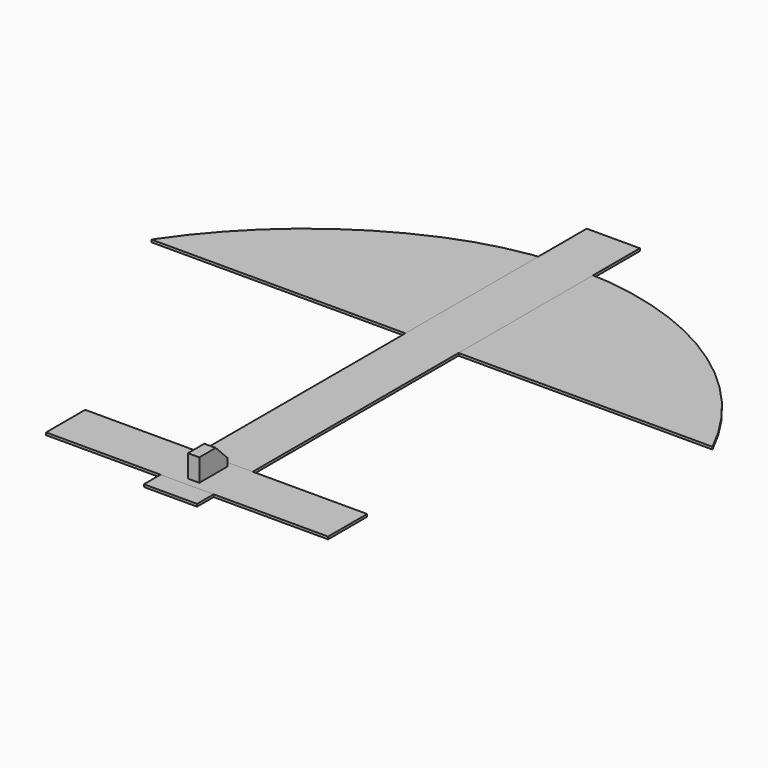
from build123d import *

# Parameters (mm, degrees)
F0_W        = 143.0713832378
F0_H        = 45.0311638415
F4_DEPTH    = 0.635
F3_W        = 2.8990160208
F3_H        = 9.0372115374
F5_DEPTH    = 6.35
F1_W        = 13.562570326
F1_H        = 141.1334902227
F6_DEPTH    = 0.635
F2_W        = 33.8059067726
F2_H        = 12.464389205
F7_T1_DEPTH = 422.6103184628
F8_T1_DEPTH = 494.0274907259
F9_SIZE     = 3.81
F10_DEPTH   = 19.05
F11_DEPTH   = 19.05


# Not quite as in the source:
# - a fillet or chamfer that OpenCascade refuses, or shapes differently, is made with other operations: its cross-section is extruded or revolved along the edge and cut away or added


with BuildPart() as f4:
    # F0 (on Top) → F4 (new body)
    with BuildSketch(Plane.XY):
        Rectangle(F0_W, F0_H)
    extrude(amount=F4_DEPTH)

    # F7: fillet of radius 101.6 on 1 edges, made by hand

    # F7_s2 → F7_t1 (cut)
    with BuildSketch(Plane.XY.offset(-210.9876592314)):
        with BuildLine():
            ThreePointArc((12.8593720736, 22.5155819207), (-34.969313076, 10.5536144563), (-71.5356916189, -22.5155819207))
            Line((-71.5356916189, -22.5155819207), (-71.5356916189, 22.5155819207))
            Line((-71.5356916189, 22.5155819207), (12.8593720736, 22.5155819207))
        make_face()
    extrude(amount=F7_T1_DEPTH, mode=Mode.SUBTRACT)

    # F8: fillet of radius 76.2 on 1 edges, made by hand

    # F8_s2 → F8_t1 (cut)
    with BuildSketch(Plane.XY.offset(-246.696245363)):
        with BuildLine():
            ThreePointArc((71.5356916189, -22.5155819207), (29.7510071905, 15.6271915076), (-26.8126321644, 14.4500252009))
            Line((-26.8126321644, 14.4500252009), (-29.7880324822, 21.4651084469))
            ThreePointArc((-29.7880324822, 21.4651084469), (12.8593720736, 30.1355819207), (71.5356916189, 30.1355819207))
            Line((71.5356916189, 30.1355819207), (79.1556916189, 22.5155819207))
            ThreePointArc((79.1556916189, 22.5155819207), (79.1556916189, 0), (78.3951236794, -19.1970593869))
            Line((78.3951236794, -19.1970593869), (71.5356916189, -22.5155819207))
        make_face()
    extrude(amount=F8_T1_DEPTH, mode=Mode.SUBTRACT)


with BuildPart() as f5:
    # F3 (on Top) → F5 (new body)
    with BuildSketch(Plane.XY):
        with Locations((0, -93.9688310027)):
            Rectangle(F3_W, F3_H)
    extrude(amount=F5_DEPTH)

    # F9
    f9_edges = [f5.edges().sort_by_distance(p)[0] for p in [
        (0, -89.450225, 6.35),
    ]]
    chamfer(f9_edges, length=F9_SIZE)


with BuildPart() as f6:
    # F1 (on Top) → F6 (new body)
    with BuildSketch(Plane.XY):
        with Locations((0, -35.2845847517)):
            Rectangle(F1_W, F1_H)
    extrude(amount=F6_DEPTH)


with BuildPart() as f6b:
    # F2 (on Top) → F6, piece 2 (new body)
    with BuildSketch(Plane.XY):
        with Locations((0, -94.3314284086)):
            Rectangle(F2_W, F2_H)
    extrude(amount=F6_DEPTH)

    # F10 (add): a face of the model
    f10_faces = [f6b.faces().sort_by_distance(p)[0] for p in [
        (-16.9029533863, -94.3314284086, 0.3175),
    ]]
    extrude(f10_faces, amount=F10_DEPTH)

    # F11 (add): a face of the model
    f11_faces = [f6b.faces().sort_by_distance(p)[0] for p in [
        (16.9029533863, -94.3314284086, 0.3175),
    ]]
    extrude(f11_faces, amount=F11_DEPTH)


solid = Compound([f4.part, f5.part, f6.part, f6b.part])
